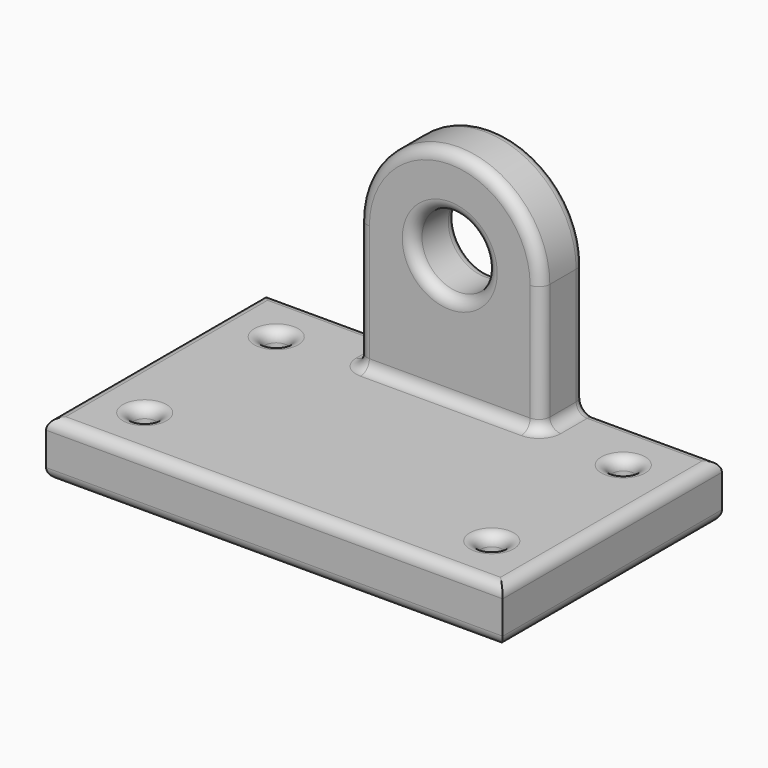
from build123d import *

# Parameters (mm, degrees)
F0_W     = 125
F0_H     = 75
F1_DEPTH = 15
F2_W     = 50
F2_H     = 15
F3_DEPTH = 15
F4_R     = 3
F5_DEPTH = 25
F6_R     = 3


with BuildPart() as f1:
    # F0 (on Top) → F1 (new body)
    with BuildSketch(Plane.XY):
        Rectangle(F0_W, F0_H)
    extrude(amount=F1_DEPTH)

    # F2 (on face) → F3 (join)
    with BuildSketch(Plane(origin=(0, 37.5, 0), x_dir=(-1, 0, 0), z_dir=(0, 1, 0))):
        with BuildLine():
            Line((10, 50), (25, 50))
            ThreePointArc((25, 50), (0, 75), (-25, 50))
            Line((-25, 50), (-10, 50))
            ThreePointArc((-10, 50), (0, 60), (10, 50))
        make_face()
        with BuildLine():
            ThreePointArc((-25, 50), (0, 25), (25, 50))
            Line((25, 50), (10, 50))
            ThreePointArc((10, 50), (0, 40), (-10, 50))
            Line((-10, 50), (-25, 50))
        make_face()
        with BuildLine():
            Line((25, 15), (25, 50))
            ThreePointArc((25, 50), (0, 25), (-25, 50))
            Line((-25, 50), (-25, 15))
            Line((-25, 15), (25, 15))
        make_face()
        with Locations((0, 7.5)):
            Rectangle(F2_W, F2_H)
    extrude(amount=-F3_DEPTH)

    # F4 (on face) → F5 (cut)
    with BuildSketch(Plane.XY.offset(15)):
        with Locations((-47.5, 22.5)):
            Circle(F4_R)
        with Locations((-47.5, -22.5)):
            Circle(F4_R)
        with Locations((47.5, -22.5)):
            Circle(F4_R)
        with Locations((47.5, 22.5)):
            Circle(F4_R)
    extrude(amount=-F5_DEPTH, mode=Mode.SUBTRACT)

    # F6
    f6_edges = [f1.edges().sort_by_distance(p)[0] for p in [
        (-25, 22.5, 32.5),
        (0, 22.5, 15),
        (25, 22.5, 32.5),
        (0, 22.5, 75),
        (10, 22.5, 50),
        (0, 37.5, 0),
        (0, -37.5, 15),
        (-62.5, 0, 15),
        (62.5, 0, 15),
        (-43.75, 37.5, 15),
        (43.75, 37.5, 15),
        (-25, 30, 15),
        (25, 30, 15),
        (-50.5, -22.5, 15),
        (44.5, -22.5, 15),
        (-50.5, 22.5, 15),
        (44.5, 22.5, 15),
        (0, -37.5, 0),
        (-62.5, 0, 0),
        (62.5, 0, 0),
        (-50.5, -22.5, 0),
        (44.5, -22.5, 0),
        (-50.5, 22.5, 0),
        (44.5, 22.5, 0),
        (10, 37.5, 50),
        (25, 37.5, 32.5),
        (0, 37.5, 75),
        (-25, 37.5, 32.5),
    ]]
    fillet(f6_edges, radius=F6_R)


solid = f1.part
